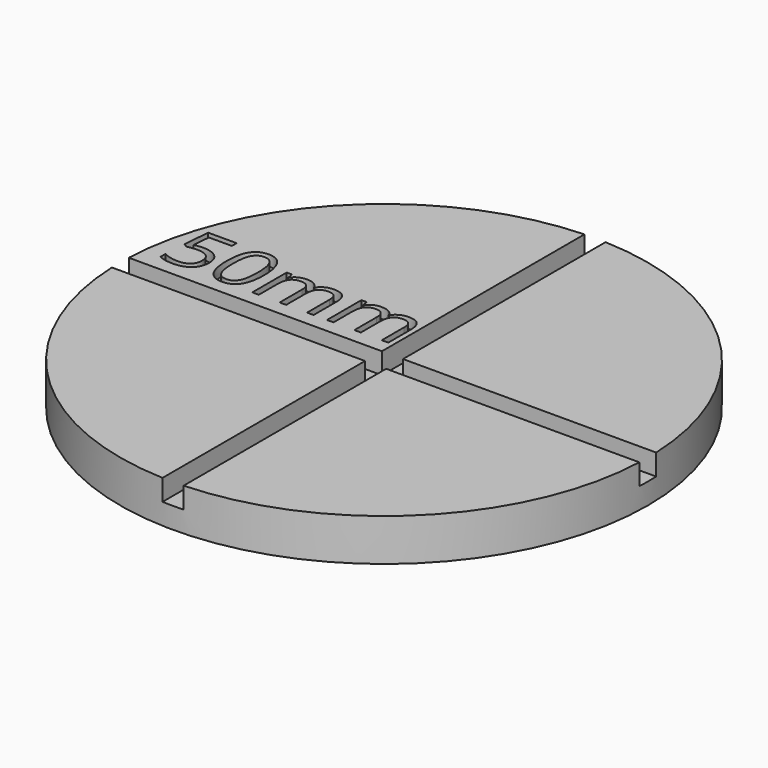
from build123d import *

# Parameters (mm, degrees)
F0_R         = 25
F1_DEPTH     = 4
F2_W         = 24
F2_H         = 2
F2_W_2       = 2
F2_H_2       = 24
F3_DEPTH     = 2
F4_TEXT_SIZE = 7.6100456336
F5_DEPTH     = 1


# Not quite as in the source:
# - Text() gives the source's letters only with a copy of the font that has no kerning and outlines rounded to 1/6400 em; it was checked with that copy


with BuildPart() as f1:
    # F0 (on Top) → F1 (new body)
    with BuildSketch(Plane.XY):
        Circle(F0_R)
    extrude(amount=F1_DEPTH)

    # F2 (on face) → F3 (cut)
    with BuildSketch(Plane.XY.offset(4)):
        with Locations((13, 0)):
            Rectangle(F2_W, F2_H)
        with Locations((0, -13)):
            Rectangle(F2_W_2, F2_H_2)
        Rectangle(F2_W_2, F2_H)
        with Locations((-13, 0)):
            Rectangle(F2_W, F2_H)
        with Locations((0, 13)):
            Rectangle(F2_W_2, F2_H_2)
    extrude(amount=-F3_DEPTH, mode=Mode.SUBTRACT)

    # F4 (on face) → F5 (cut)
    with BuildSketch(Plane.XY.offset(4)):
        with Locations((-23.7350113302, 2.3724699626)):
            Text('50mm', F4_TEXT_SIZE, font='Open Sans', text_align=(TextAlign.LEFT, TextAlign.BOTTOM))
    extrude(amount=-F5_DEPTH, mode=Mode.SUBTRACT)


solid = f1.part
